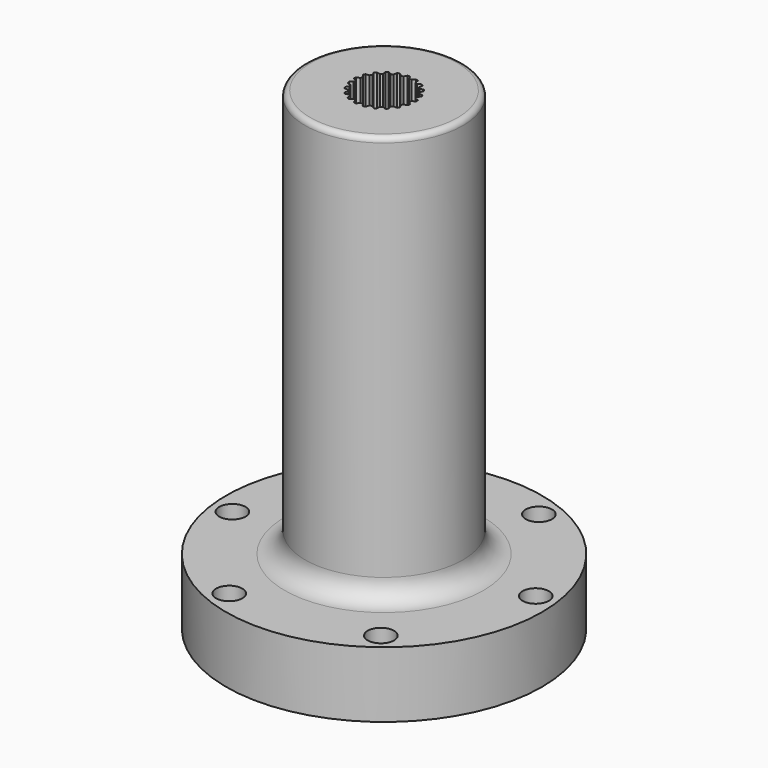
from build123d import *

# Parameters (mm, degrees)
F3_DEPTH = 145
F4_R     = 45
F4_R_2   = 40
F5_DEPTH = 5
F6_R     = 5
F7_DEPTH = 63.7
F8_R     = 7.7254833996
F9_R     = 2
F10_SIZE = 1


with BuildPart() as f1:
    # F0 (on Front) → F1 (revolve)
    with BuildSketch(Plane.XZ):
        Polygon((289.0219837427, -43.7800835492), (259.0219837427, -43.7800835492), (259.0219837427, -223.7800835492), (319.0219837427, -223.7800835492), (319.0219837427, -198.7800835492), (289.0219837427, -198.7800835492), align=None)
    revolve(axis=Axis((259.0219837427, 0, -133.7800835492), (0, 0, -1)))

    # F2 (on face) → F3 (cut)
    with BuildSketch(Plane.XY.offset(-43.7800835492)):
        with BuildLine():
            Line((265.8861714025, 8.1035379787), (266.0771667967, 9.4959618826))
            ThreePointArc((266.0771667967, 9.4959618826), (265.6860600296, 9.7744047002), (265.2839775733, 10.0367491383))
            Line((265.2839775733, 10.0367491383), (264.0575851671, 9.3502469644))
            ThreePointArc((264.0575851671, 9.3502469644), (265.0044427593, 8.7746557832), (265.8861714025, 8.1035379787))
        make_face()
        with BuildLine():
            Line((269.5655949679, -1.2714803706), (269.6373358577, -0.3141647253))
            ThreePointArc((269.6373358577, -0.3141647253), (269.6408217079, -0.1570995524), (269.6419837427, 0))
            ThreePointArc((269.6419837427, 0), (269.599389219, 0.9502070251), (269.4719473226, 1.8927919004))
            Line((269.4719473226, 1.8927919004), (269.258327226, 2.8287226961))
            ThreePointArc((269.258327226, 2.8287226961), (268.9078629533, 3.8799216788), (268.4497745544, 4.8888813046))
            Line((268.4497745544, 4.8888813046), (267.9697745544, 5.7202656922))
            ThreePointArc((267.9697745544, 5.7202656922), (267.3250340865, 6.6214616957), (266.5899011994, 7.4505721504))
            Line((266.5899011994, 7.4505721504), (265.8861714025, 8.1035379787))
            ThreePointArc((265.8861714025, 8.1035379787), (265.0044427593, 8.7746557832), (264.0575851671, 9.3502469644))
            Line((264.0575851671, 9.3502469644), (263.1926550539, 9.7667753539))
            ThreePointArc((263.1926550539, 9.7667753539), (262.152283695, 10.1481831974), (261.0778338499, 10.4191113026))
            Line((261.0778338499, 10.4191113026), (260.1285562567, 10.5621918782))
            ThreePointArc((260.1285562567, 10.5621918782), (259.0219837427, 10.62), (257.9154112287, 10.5621918782))
            Line((257.9154112287, 10.5621918782), (256.9661336355, 10.4191113026))
            ThreePointArc((256.9661336355, 10.4191113026), (255.8916837905, 10.1481831974), (254.8513124315, 9.7667753539))
            Line((254.8513124315, 9.7667753539), (253.9863823183, 9.3502469644))
            ThreePointArc((253.9863823183, 9.3502469644), (253.0395247261, 8.7746557832), (252.157796083, 8.1035379787))
            Line((252.157796083, 8.1035379787), (251.454066286, 7.4505721504))
            ThreePointArc((251.454066286, 7.4505721504), (250.7189333989, 6.6214616957), (250.074192931, 5.7202656922))
            Line((250.074192931, 5.7202656922), (249.594192931, 4.8888813046))
            ThreePointArc((249.594192931, 4.8888813046), (249.1361045321, 3.8799216788), (248.7856402594, 2.8287226961))
            Line((248.7856402594, 2.8287226961), (248.5720201628, 1.8927919004))
            ThreePointArc((248.5720201628, 1.8927919004), (248.4316794166, 0.7936335939), (248.4066316277, -0.3141647253))
            Line((248.4066316277, -0.3141647253), (248.4783725176, -1.2714803706))
            ThreePointArc((248.4783725176, -1.2714803706), (248.6682493153, -2.3631723186), (248.9708436162, -3.4291372321))
            Line((248.9708436162, -3.4291372321), (249.3215709996, -4.3227760308))
            ThreePointArc((249.3215709996, -4.3227760308), (249.8247939545, -5.31), (250.4281435136, -6.2394158473))
            Line((250.4281435136, -6.2394158473), (251.0266937234, -6.9899740705))
            ThreePointArc((251.0266937234, -6.9899740705), (251.7985492676, -7.7850108788), (252.6490438288, -8.4952949833))
            Line((252.6490438288, -8.4952949833), (253.4422330521, -9.0360822391))
            ThreePointArc((253.4422330521, -9.0360822391), (254.4141384333, -9.5682893771), (255.4362078225, -9.996329879))
            Line((255.4362078225, -9.996329879), (256.3535577161, -10.2792948465))
            ThreePointArc((256.3535577161, -10.2792948465), (257.4391548759, -10.5013833745), (258.5419837427, -10.6091469968))
            Line((258.5419837427, -10.6091469968), (259.5019837427, -10.6091469968))
            ThreePointArc((259.5019837427, -10.6091469968), (260.6048126095, -10.5013833745), (261.6904097693, -10.2792948465))
            Line((261.6904097693, -10.2792948465), (262.6077596629, -9.996329879))
            ThreePointArc((262.6077596629, -9.996329879), (263.6298290521, -9.5682893771), (264.6017344333, -9.0360822391))
            Line((264.6017344333, -9.0360822391), (265.3949236566, -8.4952949833))
            ThreePointArc((265.3949236566, -8.4952949833), (266.2454182178, -7.7850108788), (267.0172737621, -6.9899740705))
            Line((267.0172737621, -6.9899740705), (267.6158239718, -6.2394158473))
            ThreePointArc((267.6158239718, -6.2394158473), (268.2191735309, -5.31), (268.7223964859, -4.3227760308))
            Line((268.7223964859, -4.3227760308), (269.0731238693, -3.4291372321))
            ThreePointArc((269.0731238693, -3.4291372321), (269.3757181701, -2.3631723186), (269.5655949679, -1.2714803706))
        make_face()
        with BuildLine():
            Line((263.1926550539, 9.7667753539), (262.964740908, 11.1536346513))
            ThreePointArc((262.964740908, 11.1536346513), (262.508937456, 11.3044262925), (262.0473910145, 11.4365996188))
            Line((262.0473910145, 11.4365996188), (261.0778338499, 10.4191113026))
            ThreePointArc((261.0778338499, 10.4191113026), (262.152283695, 10.1481831974), (263.1926550539, 9.7667753539))
        make_face()
        with BuildLine():
            Line((260.1285562567, 10.5621918782), (259.5019837427, 11.8202580344))
            ThreePointArc((259.5019837427, 11.8202580344), (259.0219837427, 11.83), (258.5419837427, 11.8202580344))
            Line((258.5419837427, 11.8202580344), (257.9154112287, 10.5621918782))
            ThreePointArc((257.9154112287, 10.5621918782), (259.0219837427, 10.62), (260.1285562567, 10.5621918782))
        make_face()
        with BuildLine():
            Line((256.9661336355, 10.4191113026), (255.996576471, 11.4365996188))
            ThreePointArc((255.996576471, 11.4365996188), (255.5350300294, 11.3044262925), (255.0792265774, 11.1536346513))
            Line((255.0792265774, 11.1536346513), (254.8513124315, 9.7667753539))
            ThreePointArc((254.8513124315, 9.7667753539), (255.8916837905, 10.1481831974), (256.9661336355, 10.4191113026))
        make_face()
        with BuildLine():
            Line((253.9863823183, 9.3502469644), (252.7599899121, 10.0367491383))
            ThreePointArc((252.7599899121, 10.0367491383), (252.3579074558, 9.7744047002), (251.9668006888, 9.4959618826))
            Line((251.9668006888, 9.4959618826), (252.157796083, 8.1035379787))
            ThreePointArc((252.157796083, 8.1035379787), (253.0395247261, 8.7746557832), (253.9863823183, 9.3502469644))
        make_face()
        with BuildLine():
            Line((251.454066286, 7.4505721504), (250.0798089854, 7.7450894514))
            ThreePointArc((250.0798089854, 7.7450894514), (249.7729173051, 7.375884356), (249.4812587756, 6.9945312282))
            Line((249.4812587756, 6.9945312282), (250.074192931, 5.7202656922))
            ThreePointArc((250.074192931, 5.7202656922), (250.7189333989, 6.6214616957), (251.454066286, 7.4505721504))
        make_face()
        with BuildLine():
            Line((249.594192931, 4.8888813046), (248.194179528, 4.7652445779))
            ThreePointArc((248.194179528, 4.7652445779), (248.0097472963, 4.3219843183), (247.8434521446, 3.8716057792))
            Line((247.8434521446, 3.8716057792), (248.7856402594, 2.8287226961))
            ThreePointArc((248.7856402594, 2.8287226961), (249.1361045321, 3.8799216788), (249.594192931, 4.8888813046))
        make_face()
        with BuildLine():
            Line((248.5720201628, 1.8927919004), (247.2706479921, 1.3619868118))
            ThreePointArc((247.2706479921, 1.3619868118), (247.2250628221, 0.8840570071), (247.1989071022, 0.4046711665))
            Line((247.1989071022, 0.4046711665), (248.4066316277, -0.3141647253))
            ThreePointArc((248.4066316277, -0.3141647253), (248.4316794166, 0.7936335939), (248.5720201628, 1.8927919004))
        make_face()
        with BuildLine():
            ThreePointArc((247.3912742075, -2.1622894596), (247.4885865416, -2.6324226487), (247.6048943041, -3.0982202553))
            Line((247.6048943041, -3.0982202553), (248.9708436162, -3.4291372321))
            ThreePointArc((248.9708436162, -3.4291372321), (248.6682493153, -2.3631723186), (248.4783725176, -1.2714803706))
            Line((248.4783725176, -1.2714803706), (247.3912742075, -2.1622894596))
        make_face()
        with BuildLine():
            ThreePointArc((248.5453400056, -5.4944368234), (248.7769032159, -5.915), (249.0253400056, -6.325821211))
            Line((249.0253400056, -6.325821211), (250.4281435136, -6.2394158473))
            ThreePointArc((250.4281435136, -6.2394158473), (249.8247939545, -5.31), (249.3215709996, -4.3227760308))
            Line((249.3215709996, -4.3227760308), (248.5453400056, -5.4944368234))
        make_face()
        with BuildLine():
            ThreePointArc((250.6303015758, -8.3383793635), (250.9755402549, -8.6720036437), (251.3340313728, -8.9913451918))
            Line((251.3340313728, -8.9913451918), (252.6490438288, -8.4952949833))
            ThreePointArc((252.6490438288, -8.4952949833), (251.7985492676, -7.7850108788), (251.0266937234, -6.9899740705))
            Line((251.0266937234, -6.9899740705), (250.6303015758, -8.3383793635))
        make_face()
        with BuildLine():
            ThreePointArc((253.4609009328, -10.4414203048), (253.889139109, -10.6584617073), (254.325831046, -10.8579486944))
            Line((254.325831046, -10.8579486944), (255.4362078225, -9.996329879))
            ThreePointArc((255.4362078225, -9.996329879), (254.4141384333, -9.5682893771), (253.4422330521, -9.0360822391))
            Line((253.4422330521, -9.0360822391), (253.4609009328, -10.4414203048))
        make_face()
        with BuildLine():
            ThreePointArc((256.7856269019, -11.6166952306), (257.2588137338, -11.6978686742), (257.7349044951, -11.7597758061))
            Line((257.7349044951, -11.7597758061), (258.5419837427, -10.6091469968))
            ThreePointArc((258.5419837427, -10.6091469968), (257.4391548759, -10.5013833745), (256.3535577161, -10.2792948465))
            Line((256.3535577161, -10.2792948465), (256.7856269019, -11.6166952306))
        make_face()
        with BuildLine():
            ThreePointArc((260.3090629904, -11.7597758061), (260.7851537516, -11.6978686742), (261.2583405835, -11.6166952306))
            Line((261.2583405835, -11.6166952306), (261.6904097693, -10.2792948465))
            ThreePointArc((261.6904097693, -10.2792948465), (260.6048126095, -10.5013833745), (259.5019837427, -10.6091469968))
            Line((259.5019837427, -10.6091469968), (260.3090629904, -11.7597758061))
        make_face()
        with BuildLine():
            ThreePointArc((263.7181364394, -10.8579486944), (264.1548283765, -10.6584617073), (264.5830665526, -10.4414203048))
            Line((264.5830665526, -10.4414203048), (264.6017344333, -9.0360822391))
            ThreePointArc((264.6017344333, -9.0360822391), (263.6298290521, -9.5682893771), (262.6077596629, -9.996329879))
            Line((262.6077596629, -9.996329879), (263.7181364394, -10.8579486944))
        make_face()
        with BuildLine():
            ThreePointArc((266.7099361127, -8.9913451918), (267.0684272305, -8.6720036437), (267.4136659096, -8.3383793635))
            Line((267.4136659096, -8.3383793635), (267.0172737621, -6.9899740705))
            ThreePointArc((267.0172737621, -6.9899740705), (266.2454182178, -7.7850108788), (265.3949236566, -8.4952949833))
            Line((265.3949236566, -8.4952949833), (266.7099361127, -8.9913451918))
        make_face()
        with BuildLine():
            ThreePointArc((269.0186274798, -6.325821211), (269.2670642695, -5.915), (269.4986274798, -5.4944368234))
            Line((269.4986274798, -5.4944368234), (268.7223964859, -4.3227760308))
            ThreePointArc((268.7223964859, -4.3227760308), (268.2191735309, -5.31), (267.6158239718, -6.2394158473))
            Line((267.6158239718, -6.2394158473), (269.0186274798, -6.325821211))
        make_face()
        with BuildLine():
            ThreePointArc((270.4390731814, -3.0982202553), (270.5553809438, -2.6324226487), (270.6526932779, -2.1622894596))
            Line((270.6526932779, -2.1622894596), (269.5655949679, -1.2714803706))
            ThreePointArc((269.5655949679, -1.2714803706), (269.3757181701, -2.3631723186), (269.0731238693, -3.4291372321))
            Line((269.0731238693, -3.4291372321), (270.4390731814, -3.0982202553))
        make_face()
        with BuildLine():
            Line((269.6373358577, -0.3141647253), (270.8450603832, 0.4046711665))
            ThreePointArc((270.8450603832, 0.4046711665), (270.8189046634, 0.8840570071), (270.7733194934, 1.3619868118))
            Line((270.7733194934, 1.3619868118), (269.4719473226, 1.8927919004))
            ThreePointArc((269.4719473226, 1.8927919004), (269.599389219, 0.9502070251), (269.6419837427, 0))
            ThreePointArc((269.6419837427, 0), (269.6408217079, -0.1570995524), (269.6373358577, -0.3141647253))
        make_face()
        with BuildLine():
            Line((269.258327226, 2.8287226961), (270.2005153408, 3.8716057792))
            ThreePointArc((270.2005153408, 3.8716057792), (270.0342201892, 4.3219843183), (269.8497879574, 4.7652445779))
            Line((269.8497879574, 4.7652445779), (268.4497745544, 4.8888813046))
            ThreePointArc((268.4497745544, 4.8888813046), (268.9078629533, 3.8799216788), (269.258327226, 2.8287226961))
        make_face()
        with BuildLine():
            Line((267.9697745544, 5.7202656922), (268.5627087098, 6.9945312282))
            ThreePointArc((268.5627087098, 6.9945312282), (268.2710501803, 7.375884356), (267.9641585, 7.7450894514))
            Line((267.9641585, 7.7450894514), (266.5899011994, 7.4505721504))
            ThreePointArc((266.5899011994, 7.4505721504), (267.3250340865, 6.6214616957), (267.9697745544, 5.7202656922))
        make_face()
    extrude(amount=-F3_DEPTH, mode=Mode.SUBTRACT)

    # F4 (on face) → F5 (join)
    with BuildSketch(Plane(origin=(0, 0, -223.7800835492), x_dir=(1, 0, 0), z_dir=(0, 0, -1))):
        with Locations((259.0219837427, 0)):
            Circle(F4_R)
        with Locations((259.0219837427, 0)):
            Circle(F4_R_2, mode=Mode.SUBTRACT)
    extrude(amount=F5_DEPTH)

    # F6 (on face) → F7 (cut)
    with BuildSketch(Plane.XY.offset(-198.7800835492)):
        with Locations((206.986505863, -6.968431806)):
            Circle(F6_R)
        with Locations((226.9694058344, 41.5798298389)):
            Circle(F6_R)
        with Locations((311.0574616224, 6.968431806)):
            Circle(F6_R)
        with Locations((291.0745616511, -41.5798298389)):
            Circle(F6_R)
        with Locations((239.0390837714, -48.5482616448)):
            Circle(F6_R)
        with Locations((279.004883714, 48.5482616448)):
            Circle(F6_R)
    extrude(amount=-F7_DEPTH, mode=Mode.SUBTRACT)

    # F8
    f8_edges = [f1.edges().sort_by_distance(p)[0] for p in [
        (229.021984, 0, -198.780084),
    ]]
    fillet(f8_edges, radius=F8_R)

    # F9
    f9_edges = [f1.edges().sort_by_distance(p)[0] for p in [
        (229.021984, 0, -43.780084),
    ]]
    fillet(f9_edges, radius=F9_R)

    # F10
    f10_edges = [f1.edges().sort_by_distance(p)[0] for p in [
        (214.021984, 0, -228.780084),
    ]]
    chamfer(f10_edges, length=F10_SIZE)


solid = f1.part
